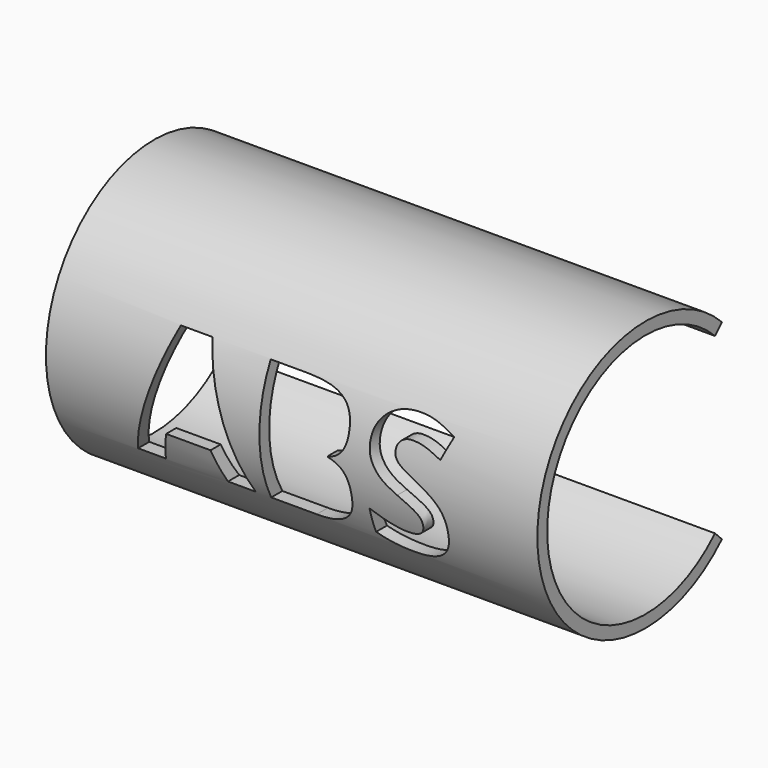
from build123d import *

# Parameters (mm, degrees)
F1_DEPTH     = 50.8
F3_TEXT_SIZE = 17.6388888889
F4_DEPTH     = 35.2792817332


# Not quite as in the source:
# - Text() gives the source's letters only with a copy of the font that has no kerning and outlines rounded to 1/6400 em; it was checked with that copy


with BuildPart() as f1:
    # F0 (on Right) → F1 (new body)
    with BuildSketch(Plane.YZ):
        with BuildLine():
            ThreePointArc((8.9802561211, -8.9802561211), (-12.7, 0), (8.9802561211, 8.9802561211))
            Line((8.9802561211, 8.9802561211), (9.8782817332, 9.8782817332))
            ThreePointArc((9.8782817332, 9.8782817332), (-13.97, 0), (9.8782817332, -9.8782817332))
            Line((9.8782817332, -9.8782817332), (8.9802561211, -8.9802561211))
        make_face()
    extrude(amount=F1_DEPTH)

    # F3 (on offset) → F4 (cut, through all)
    with BuildSketch(Plane.XZ.offset(25.4)):
        with BuildLine():
            Line((26.3880533854, -0.8626519097), (24.7344075521, -0.8626519097))
            Line((24.7344075521, -0.8626519097), (24.7344075521, -4.1451388889))
            Line((24.7344075521, -4.1451388889), (26.4734917535, -4.1451388889))
            add(Edge.make_bspline(
                [(26.4734917535, -4.1451388889), (27.575922309, -4.1451388889), (28.1009548611, -3.7234592014)],
                knots=[0, 0, 0, 1, 1, 1], degree=2))
            add(Edge.make_bspline(
                [(28.1009548611, -3.7234592014), (28.6259874132, -3.3017795139), (28.6259874132, -2.430859375)],
                knots=[0, 0, 0, 1, 1, 1], degree=2))
            add(Edge.make_bspline(
                [(28.6259874132, -2.430859375), (28.6259874132, -0.8626519097), (26.3880533854, -0.8626519097)],
                knots=[0, 0, 0, 1, 1, 1], degree=2))
        make_face()
        with BuildLine():
            Line((24.7344075521, 4.0541883681), (24.7344075521, 1.2540147569))
            Line((24.7344075521, 1.2540147569), (26.2833224826, 1.2540147569))
            add(Edge.make_bspline(
                [(26.2833224826, 1.2540147569), (27.3692165799, 1.2540147569), (27.8556640625, 1.5902560764)],
                knots=[0, 0, 0, 1, 1, 1], degree=2))
            add(Edge.make_bspline(
                [(27.8556640625, 1.5902560764), (28.3421115451, 1.9264973958), (28.3421115451, 2.7009548611)],
                knots=[0, 0, 0, 1, 1, 1], degree=2))
            add(Edge.make_bspline(
                [(28.3421115451, 2.7009548611), (28.3421115451, 3.4258029514), (27.8129448785, 3.7399956597)],
                knots=[0, 0, 0, 1, 1, 1], degree=2))
            add(Edge.make_bspline(
                [(27.8129448785, 3.7399956597), (27.2837782118, 4.0541883681), (26.137250434, 4.0541883681)],
                knots=[0, 0, 0, 1, 1, 1], degree=2))
            Line((26.137250434, 4.0541883681), (24.7344075521, 4.0541883681))
        make_face()
        with Locations((8.3081922743, -6.35)):
            Text('ABS', F3_TEXT_SIZE, font='Open Sans', font_style=FontStyle.BOLD, text_align=(TextAlign.LEFT, TextAlign.BOTTOM))
        with BuildLine():
            Line((12.7702799479, -1.1134548611), (16.0500108507, -1.1134548611))
            add(Edge.make_bspline(
                [(16.0500108507, -1.1134548611), (14.7849717882, 2.9600260417), (14.6251193576, 3.4947048611)],
                knots=[0, 0, 0, 1, 1, 1], degree=2))
            add(Edge.make_bspline(
                [(14.6251193576, 3.4947048611), (14.4652669271, 4.0293836806), (14.3963650174, 4.3380642361)],
                knots=[0, 0, 0, 1, 1, 1], degree=2))
            add(Edge.make_bspline(
                [(14.3963650174, 4.3380642361), (14.1124891493, 3.2356336806), (12.7702799479, -1.1134548611)],
                knots=[0, 0, 0, 1, 1, 1], degree=2))
        make_face()
    extrude(amount=-F4_DEPTH, mode=Mode.SUBTRACT)


solid = f1.part
